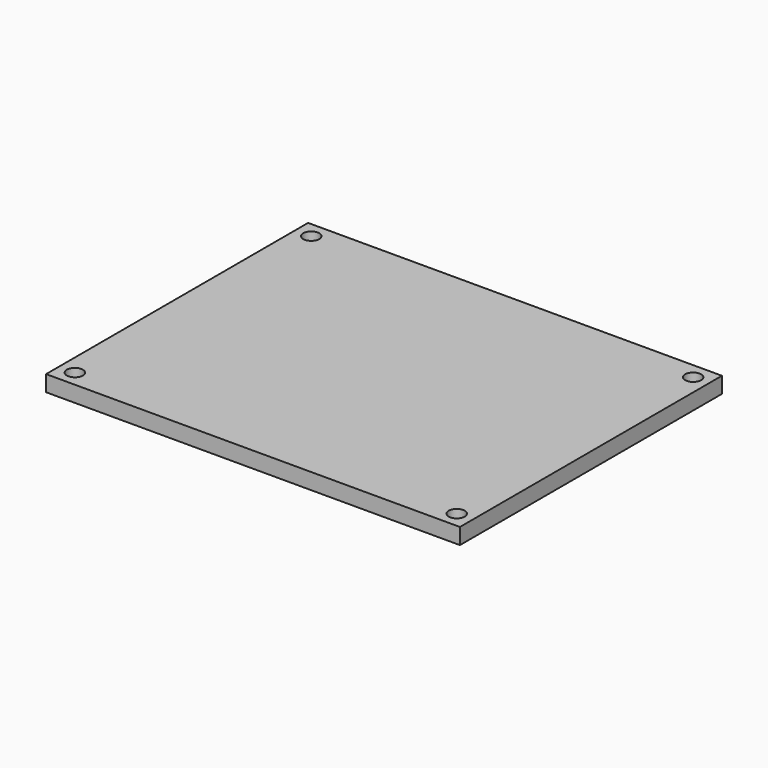
from build123d import *

# Parameters (mm, degrees)
F0_W     = 82.169
F0_H     = 65.024
F1_DEPTH = 3.175
F2_R     = 1.5875
F3_DEPTH = 25.4


# Not quite as in the source:
# - a pattern or mirror of a feature is missing from the dataset's text; its kind, count and spacing are read off the source's solid


with BuildPart() as f1:
    # F0 (on Top) → F1 (new body)
    with BuildSketch(Plane.XY):
        Rectangle(F0_W, F0_H)
    extrude(amount=F1_DEPTH)

    # F2 (on face) → F3 (cut)
    with BuildSketch(Plane.XY.offset(3.175)):
        with Locations((-37.9095, 29.337)):
            Circle(F2_R)
    f3 = extrude(amount=-F3_DEPTH, mode=Mode.SUBTRACT)

    # F3_copies: F3 across plane
    add(f3.mirror(Plane(origin=(0, 0, 0), x_dir=(0, 0, 1), z_dir=(1, 0, 0))), mode=Mode.SUBTRACT)

    # F3_copies1: F3 across plane
    add(f3.mirror(Plane(origin=(0, 0, 0), x_dir=(0, 0, -1), z_dir=(0, -1, 0))), mode=Mode.SUBTRACT)

    # F3_copies2: F3 across plane
    add(f3.mirror(Plane(origin=(0, 0, 0), x_dir=(0.6120128715, 0.7908478015, 0), z_dir=(0.7908478015, -0.6120128715, 0))), mode=Mode.SUBTRACT)


solid = f1.part
